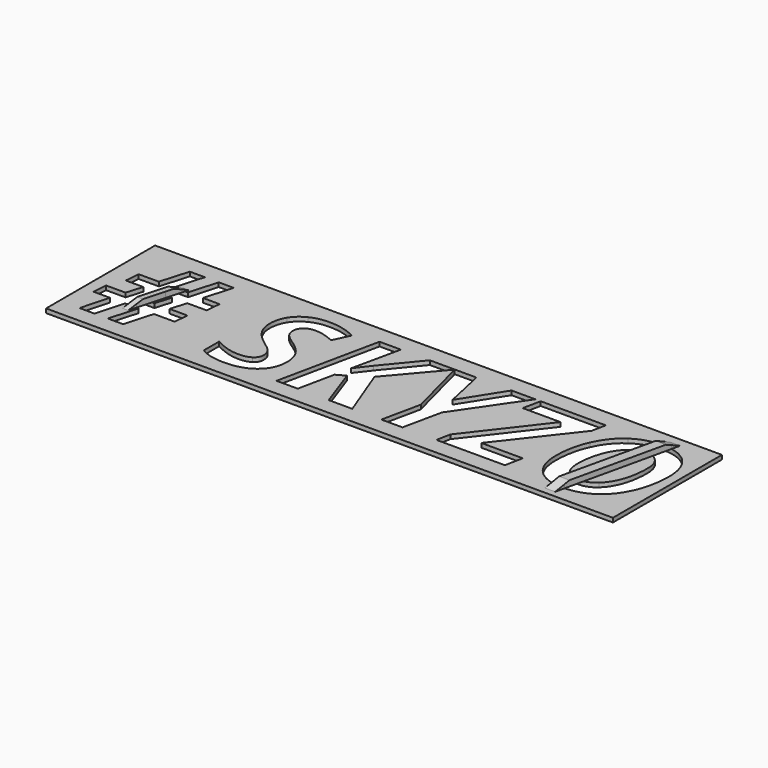
from build123d import *

# Parameters (mm, degrees)
F0_W       = 203
F0_H       = 48.8051118211
F1_DEPTH   = 1.5
F3_DEPTH   = 2
F4_SIZE2   = 1.99999
F4_SIZE    = 4.99999
F4_2_SIZE2 = 1.99999
F4_2_SIZE  = 4.99999


# Not quite as in the source:
# - a fillet or chamfer is up to 0.001 mm smaller than in the source, because OpenCascade refuses the exact size


with BuildPart() as f1:
    # F0 (on Top) → F1 (new body)
    with BuildSketch(Plane.XY):
        with Locations((-1.5, -1.4213357481)):
            Rectangle(F0_W, F0_H)
        Polygon((-67.1805111821, 1.294319204), (-74.1373801917, 1.294319204), (-75.8626198083, -4.4964156203), (-69.4249201278, -4.4964156203), (-69.8961661342, -9.6401855883), (-77.3083067093, -9.6401855883), (-80.2076677316, -19.8238916586), (-85.6948881789, -19.8238916586), (-82.7795527157, -9.6401855883), (-87.6198083067, -9.6401855883), (-90.4872204473, -19.8238916586), (-95.8546325879, -19.8238916586), (-93.03514377, -9.6401855883), (-98.9776357827, -9.6401855883), (-98.5303514377, -4.4964156203), (-91.6134185304, -4.4964156203), (-89.8642172524, 1.294319204), (-96.1581469649, 1.294319204), (-95.7028753994, 6.5099741561), (-88.4904153355, 6.5099741561), (-85.5191693291, 16.669718565), (-80.1038338658, 16.669718565), (-83.0271565495, 6.5099741561), (-78.0591054313, 6.5099741561), (-75.1677316294, 16.669718565), (-69.8003194888, 16.669718565), (-72.6916932907, 6.5099741561), (-66.7252396166, 6.5099741561), align=None, mode=Mode.SUBTRACT)
        with BuildLine():
            add(Edge.make_bspline(
                [(-31.5854632588, -3.4141472497), (-30.0878594249, -5.8222942145), (-30.0878594249, -9.0411440548)],
                knots=[0, 0, 0, 1, 1, 1], degree=2))
            add(Edge.make_bspline(
                [(-30.0878594249, -9.0411440548), (-30.0878594249, -14.2567990068), (-33.7819488818, -17.2919427768)],
                knots=[0, 0, 0, 1, 1, 1], degree=2))
            add(Edge.make_bspline(
                [(-33.7819488818, -17.2919427768), (-37.4760383387, -20.3270865468), (-43.785942492, -20.3270865468)],
                knots=[0, 0, 0, 1, 1, 1], degree=2))
            add(Edge.make_bspline(
                [(-43.785942492, -20.3270865468), (-49.3051118211, -20.3270865468), (-52.6757188498, -18.0746903806)],
                knots=[0, 0, 0, 1, 1, 1], degree=2))
            Line((-52.6757188498, -18.0746903806), (-52.6757188498, -11.2376296778))
            add(Edge.make_bspline(
                [(-52.6757188498, -11.2376296778), (-47.8594249201, -13.9293229685), (-43.7380191693, -13.9293229685)],
                knots=[0, 0, 0, 1, 1, 1], degree=2))
            add(Edge.make_bspline(
                [(-43.7380191693, -13.9293229685), (-40.9424920128, -13.9293229685), (-39.3690095847, -12.8710162592)],
                knots=[0, 0, 0, 1, 1, 1], degree=2))
            add(Edge.make_bspline(
                [(-39.3690095847, -12.8710162592), (-37.7955271565, -11.81270955), (-37.7955271565, -9.9676616267)],
                knots=[0, 0, 0, 1, 1, 1], degree=2))
            add(Edge.make_bspline(
                [(-37.7955271565, -9.9676616267), (-37.7955271565, -8.8893868663), (-38.1349840256, -8.0786839909)],
                knots=[0, 0, 0, 1, 1, 1], degree=2))
            add(Edge.make_bspline(
                [(-38.1349840256, -8.0786839909), (-38.4744408946, -7.2679811155), (-39.0974440895, -6.5690993263)],
                knots=[0, 0, 0, 1, 1, 1], degree=2))
            add(Edge.make_bspline(
                [(-39.0974440895, -6.5690993263), (-39.7204472843, -5.8702175372), (-42.1884984026, -4.0251696139)],
                knots=[0, 0, 0, 1, 1, 1], degree=2))
            add(Edge.make_bspline(
                [(-42.1884984026, -4.0251696139), (-45.6389776358, -1.5491312752), (-47.0367412141, 0.8709965203)],
                knots=[0, 0, 0, 1, 1, 1], degree=2))
            add(Edge.make_bspline(
                [(-47.0367412141, 0.8709965203), (-48.4345047923, 3.2911243158), (-48.4345047923, 6.0866514724)],
                knots=[0, 0, 0, 1, 1, 1], degree=2))
            add(Edge.make_bspline(
                [(-48.4345047923, 6.0866514724), (-48.4345047923, 9.3055013126), (-46.8849840256, 11.8374501944)],
                knots=[0, 0, 0, 1, 1, 1], degree=2))
            add(Edge.make_bspline(
                [(-46.8849840256, 11.8374501944), (-45.3354632588, 14.3693990762), (-42.4760383387, 15.7791434852)],
                knots=[0, 0, 0, 1, 1, 1], degree=2))
            add(Edge.make_bspline(
                [(-42.4760383387, 15.7791434852), (-39.6166134185, 17.1888878941), (-35.9025559105, 17.1888878941)],
                knots=[0, 0, 0, 1, 1, 1], degree=2))
            add(Edge.make_bspline(
                [(-35.9025559105, 17.1888878941), (-30.4872204473, 17.1888878941), (-25.9904153355, 14.7208367759)],
                knots=[0, 0, 0, 1, 1, 1], degree=2))
            Line((-25.9904153355, 14.7208367759), (-28.714057508, 8.9061402903))
            add(Edge.make_bspline(
                [(-28.714057508, 8.9061402903), (-32.6038338658, 10.7511882136), (-35.9025559105, 10.7511882136)],
                knots=[0, 0, 0, 1, 1, 1], degree=2))
            add(Edge.make_bspline(
                [(-35.9025559105, 10.7511882136), (-37.9712460064, 10.7511882136), (-39.2931309904, 9.6289837408)],
                knots=[0, 0, 0, 1, 1, 1], degree=2))
            add(Edge.make_bspline(
                [(-39.2931309904, 9.6289837408), (-40.6150159744, 8.5067792679), (-40.6150159744, 6.6617313446)],
                knots=[0, 0, 0, 1, 1, 1], degree=2))
            add(Edge.make_bspline(
                [(-40.6150159744, 6.6617313446), (-40.6150159744, 5.1361722392), (-39.7923322684, 4.0019869356)],
                knots=[0, 0, 0, 1, 1, 1], degree=2))
            add(Edge.make_bspline(
                [(-39.7923322684, 4.0019869356), (-38.9696485623, 2.8678016321), (-36.1022364217, 0.990804827)],
                knots=[0, 0, 0, 1, 1, 1], degree=2))
            add(Edge.make_bspline(
                [(-36.1022364217, 0.990804827), (-33.0830670927, -1.0060002848), (-31.5854632588, -3.4141472497)],
                knots=[0, 0, 0, 1, 1, 1], degree=2))
        make_face(mode=Mode.SUBTRACT)
        Polygon((-5.3993610224, -0.8063197736), (1.8690095847, -19.8238916586), (-6.5734824281, -19.8238916586), (-11.8370607029, -5.0475338311), (-14.9600638978, -6.7967351091), (-17.6757188498, -19.8238916586), (-25.2875399361, -19.8238916586), (-17.5798722045, 16.669718565), (-9.9361022364, 16.669718565), (-13.7300319489, -0.8542430963), (-9.7923322684, 4.2655652104), (0.4153354633, 16.669718565), (9.3530351438, 16.669718565), (9.4329073482, 16.669718565), (17.1405750799, 16.669718565), (20.3594249201, 1.8933607376), (29.696485623, 16.669718565), (38.2348242812, 16.669718565), (22.8115015974, -5.8702175372), (19.8402555911, -19.8238916586), (12.2763578275, -19.8238916586), (15.2476038339, -5.8702175372), (9.3718490661, 16.5977769812), align=None, mode=Mode.SUBTRACT)
        Polygon((57.8274760383, -13.4341153008), (56.5015974441, -19.8238916586), (32.0127795527, -19.8238916586), (32.9632587859, -14.8079172177), (52.3562300319, 10.2799422072), (38.8019169329, 10.2799422072), (40.1277955272, 16.669718565), (63.4904153355, 16.669718565), (62.4680511182, 11.6297824628), (42.947284345, -13.4341153008), align=None, mode=Mode.SUBTRACT)
        with BuildLine():
            add(Edge.make_bspline(
                [(93.1908945687, 13.650549236), (96.6853035144, 10.0563000347), (96.6853035144, 3.5866514724)],
                knots=[0, 0, 0, 1, 1, 1], degree=2))
            add(Edge.make_bspline(
                [(96.6853035144, 3.5866514724), (96.6853035144, -3.474051403), (94.2132587859, -9.0531248854)],
                knots=[0, 0, 0, 1, 1, 1], degree=2))
            add(Edge.make_bspline(
                [(94.2132587859, -9.0531248854), (91.7412140575, -14.6321983679), (87.4480830671, -17.4796424573)],
                knots=[0, 0, 0, 1, 1, 1], degree=2))
            add(Edge.make_bspline(
                [(87.4480830671, -17.4796424573), (83.1549520767, -20.3270865468), (77.5638977636, -20.3270865468)],
                knots=[0, 0, 0, 1, 1, 1], degree=2))
            add(Edge.make_bspline(
                [(77.5638977636, -20.3270865468), (71.1741214058, -20.3270865468), (67.5918530351, -16.6449779206)],
                knots=[0, 0, 0, 1, 1, 1], degree=2))
            add(Edge.make_bspline(
                [(67.5918530351, -16.6449779206), (64.0095846645, -12.9628692944), (64.0095846645, -6.4213357481)],
                knots=[0, 0, 0, 1, 1, 1], degree=2))
            add(Edge.make_bspline(
                [(64.0095846645, -6.4213357481), (64.0095846645, 0.1920827823), (66.481629393, 5.7471946034)],
                knots=[0, 0, 0, 1, 1, 1], degree=2))
            add(Edge.make_bspline(
                [(66.481629393, 5.7471946034), (68.9536741214, 11.3023064245), (73.2987220447, 14.2735524309)],
                knots=[0, 0, 0, 1, 1, 1], degree=2))
            add(Edge.make_bspline(
                [(73.2987220447, 14.2735524309), (77.6437699681, 17.2447984372), (83.3306709265, 17.2447984372)],
                knots=[0, 0, 0, 1, 1, 1], degree=2))
            add(Edge.make_bspline(
                [(83.3306709265, 17.2447984372), (89.696485623, 17.2447984372), (93.1908945687, 13.650549236)],
                knots=[0, 0, 0, 1, 1, 1], degree=2))
        make_face(mode=Mode.SUBTRACT)
    extrude(amount=F1_DEPTH)


with BuildPart() as f1b:
    # F0 (on Top) → F1, piece 2 (new body)
    with BuildSketch(Plane.XY):
        Polygon((-84.4488817891, 1.294319204), (-86.1980830671, -4.4964156203), (-81.2779552716, -4.4964156203), (-79.5607028754, 1.294319204), align=None)
    extrude(amount=F1_DEPTH)


with BuildPart() as f1c:
    # F0 (on Top) → F1, piece 3 (new body)
    with BuildSketch(Plane.XY):
        with BuildLine():
            add(Edge.make_bspline(
                [(87.2763578275, 8.866204188), (85.6549520767, 10.7991115363), (82.7076677316, 10.7991115363)],
                knots=[0, 0, 0, 1, 1, 1], degree=2))
            add(Edge.make_bspline(
                [(82.7076677316, 10.7991115363), (79.6884984026, 10.7991115363), (77.1685303514, 8.5187600986)],
                knots=[0, 0, 0, 1, 1, 1], degree=2))
            add(Edge.make_bspline(
                [(77.1685303514, 8.5187600986), (74.6485623003, 6.2384086609), (73.2108626198, 2.2447984372)],
                knots=[0, 0, 0, 1, 1, 1], degree=2))
            add(Edge.make_bspline(
                [(73.2108626198, 2.2447984372), (71.7731629393, -1.7488117864), (71.7731629393, -6.4213357481)],
                knots=[0, 0, 0, 1, 1, 1], degree=2))
            add(Edge.make_bspline(
                [(71.7731629393, -6.4213357481), (71.7731629393, -10.0874699334), (73.4345047923, -11.9604731282)],
                knots=[0, 0, 0, 1, 1, 1], degree=2))
            add(Edge.make_bspline(
                [(73.4345047923, -11.9604731282), (75.0958466454, -13.8334763231), (78.1150159744, -13.8334763231)],
                knots=[0, 0, 0, 1, 1, 1], degree=2))
            add(Edge.make_bspline(
                [(78.1150159744, -13.8334763231), (81.1341853035, -13.8334763231), (83.6182108626, -11.6609523615)],
                knots=[0, 0, 0, 1, 1, 1], degree=2))
            add(Edge.make_bspline(
                [(83.6182108626, -11.6609523615), (86.1022364217, -9.4884283998), (87.5, -5.5187798375)],
                knots=[0, 0, 0, 1, 1, 1], degree=2))
            add(Edge.make_bspline(
                [(87.5, -5.5187798375), (88.8977635783, -1.5491312752), (88.8977635783, 3.3869709612)],
                knots=[0, 0, 0, 1, 1, 1], degree=2))
            add(Edge.make_bspline(
                [(88.8977635783, 3.3869709612), (88.8977635783, 6.9332968398), (87.2763578275, 8.866204188)],
                knots=[0, 0, 0, 1, 1, 1], degree=2))
        make_face()
    extrude(amount=F1_DEPTH)


with BuildPart() as f3:
    # F2 (on face) → F3 (new body)
    with BuildSketch(Plane.XY.offset(1.5)):
        Polygon((-79.0633153842, 6.5099741561), (-81.1895099209, 6.5099741561), (-82.9869061708, 0), (-80.8607116342, 0), align=None)
        Polygon((-80.8607116342, 0), (-82.9869061708, 0), (-85.6485501359, -9.6401855883), (-83.5223555992, -9.6401855883), align=None)
        Polygon((-83.5223555992, -9.6401855883), (-85.6485501359, -9.6401855883), (-86.3993775221, -12.3596008982), (-84.3097966622, -12.4922116623), align=None)
        Polygon((-78.7098631263, 7.7901398763), (-80.836057663, 7.7901398763), (-81.1895099209, 6.5099741561), (-79.0633153842, 6.5099741561), align=None)
    extrude(amount=F3_DEPTH)

    # F4 (size 5 and 2 in the source; OpenCascade refuses exactly that, so slightly less here)
    f4_edges = [f3.edges().sort_by_distance(p)[0] for p in [
        (-79.77296, 7.79014, 3.5),
        (-85.354587, -12.425906, 3.5),
    ]]
    f4_side = f3.faces().sort_by_distance((-82.562621, -2.317919, 3.5))[0]
    chamfer(f4_edges, length=F4_SIZE, length2=F4_SIZE2, reference=f4_side)


with BuildPart() as f3b:
    # F2 (on face) → F3, piece 2 (new body)
    with BuildSketch(Plane.XY.offset(1.5)):
        with BuildLine():
            add(Edge.make_bspline(
                [(83.1360447097, 17.2439248851), (83.2331605644, 17.2447984372), (83.3306709265, 17.2447984372)],
                knots=[0.982853515, 0.982853515, 0.982853515, 1, 1, 1], degree=2))
            Line((83.1360447097, 17.2439248851), (74.6557232668, -20.1145648364))
            add(Edge.make_bspline(
                [(77.5638977636, -20.3270865468), (76.0287894943, -20.3270865468), (74.6557232668, -20.1145648364)],
                knots=[0, 0, 0, 0.2402444441, 0.2402444441, 0.2402444441], degree=2))
            add(Edge.make_bspline(
                [(78.3101569883, -20.3142041974), (77.9399633953, -20.3270865468), (77.5638977636, -20.3270865468)],
                knots=[0.9327379756, 0.9327379756, 0.9327379756, 1, 1, 1], degree=2))
            Line((78.3101569883, -20.3142041974), (86.7621317554, 16.9461315104))
            add(Edge.make_bspline(
                [(83.3306709265, 17.2447984372), (85.1657021856, 17.2447984372), (86.7621317554, 16.9461315104)],
                knots=[0, 0, 0, 0.2882633797, 0.2882633797, 0.2882633797], degree=2))
        make_face()
        with BuildLine():
            add(Edge.make_bspline(
                [(77.5638977636, -20.3270865468), (76.0287894943, -20.3270865468), (74.6557232668, -20.1145648364)],
                knots=[0, 0, 0, 0.2402444441, 0.2402444441, 0.2402444441], degree=2))
            Line((74.6557232668, -20.1145648364), (73.8636106253, -23.6040707678))
            Line((73.8636106253, -23.6040707678), (77.5638977636, -23.6040707678))
            Line((77.5638977636, -23.6040707678), (78.3101569883, -20.3142041974))
            add(Edge.make_bspline(
                [(78.3101569883, -20.3142041974), (77.9399633953, -20.3270865468), (77.5638977636, -20.3270865468)],
                knots=[0.9327379756, 0.9327379756, 0.9327379756, 1, 1, 1], degree=2))
        make_face()
        with BuildLine():
            Line((87.4480830671, 19.970132038), (83.754889667, 19.970132038))
            Line((83.754889667, 19.970132038), (83.1360447097, 17.2439248851))
            add(Edge.make_bspline(
                [(83.1360447097, 17.2439248851), (83.2331605644, 17.2447984372), (83.3306709265, 17.2447984372)],
                knots=[0.982853515, 0.982853515, 0.982853515, 1, 1, 1], degree=2))
            add(Edge.make_bspline(
                [(83.3306709265, 17.2447984372), (85.1657021856, 17.2447984372), (86.7621317554, 16.9461315104)],
                knots=[0, 0, 0, 0.2882633797, 0.2882633797, 0.2882633797], degree=2))
            Line((86.7621317554, 16.9461315104), (87.4480830671, 19.970132038))
        make_face()
    extrude(amount=F3_DEPTH)

    # F4#2 (size 5 and 2 in the source; OpenCascade refuses exactly that, so slightly less here)
    f4_2_edges = [f3b.edges().sort_by_distance(p)[0] for p in [
        (75.713754, -23.604071, 3.5),
        (85.601486, 19.970132, 3.5),
    ]]
    f4_2_side = f3b.faces().sort_by_distance((80.656039, -1.823937, 3.5))[0]
    chamfer(f4_2_edges, length=F4_2_SIZE, length2=F4_2_SIZE2, reference=f4_2_side)


solid = Compound([f1.part, f1b.part, f1c.part, f3.part, f3b.part])
